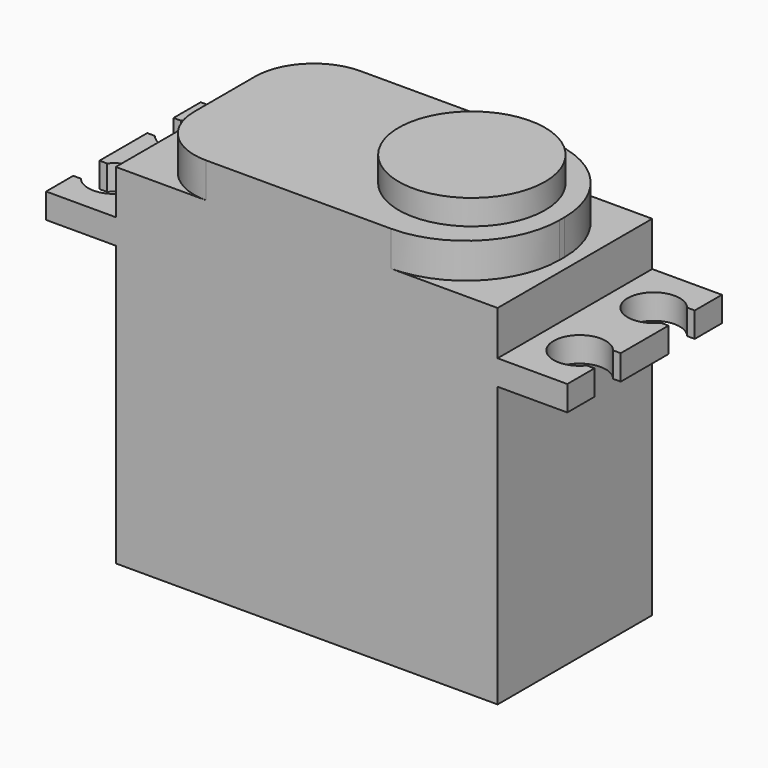
from build123d import *

# Parameters (mm, degrees)
F0_W      = 32.6
F0_H      = 29.8
F1_DEPTH  = 16.5
F2_W      = 28.8
F2_H      = 16.5
F3_DEPTH  = 3
F4_R      = 8
F5_R      = 5
F6_R      = 6.25
F7_DEPTH  = 2.14
F8_W      = 16.5
F8_H      = 2.14
F9_DEPTH  = 5.95
F11_DEPTH = 26.021


# Not quite as in the source:
# - a pattern or mirror of a feature is missing from the dataset's text; its kind, count and spacing are read off the source's solid


with BuildPart() as f1:
    # F0 (on Front) → F1 (new body)
    with BuildSketch(Plane.XZ):
        Rectangle(F0_W, F0_H)
    extrude(amount=F1_DEPTH)

    # F2 (on face) → F3 (join)
    with BuildSketch(Plane.XY.offset(14.9)):
        with Locations((0.8, -8.25)):
            Rectangle(F2_W, F2_H)
    extrude(amount=F3_DEPTH)

    # F4
    f4_edges = [f1.edges().sort_by_distance(p)[0] for p in [
        (15.2, -16.5, 16.4),
        (15.2, 0, 16.4),
    ]]
    fillet(f4_edges, radius=F4_R)

    # F5
    f5_edges = [f1.edges().sort_by_distance(p)[0] for p in [
        (-13.6, -16.5, 16.4),
        (-13.6, 0, 16.4),
    ]]
    fillet(f5_edges, radius=F5_R)

    # F6 (on face) → F7 (join)
    with BuildSketch(Plane.XY.offset(17.9)):
        with Locations((7.3, -8)):
            Circle(F6_R)
    extrude(amount=F7_DEPTH)

    # F8 (on face) → F9 (join)
    with BuildSketch(Plane.YZ.offset(16.3)):
        with Locations((-8.25, 10.05)):
            Rectangle(F8_W, F8_H)
    f9 = extrude(amount=F9_DEPTH)

    # F9_copies: F9 across plane
    add(f9.mirror(Plane(origin=(0, 0, 0), x_dir=(0, 0, -1), z_dir=(-1, 0, 0))))

    # F10 (on face) → F11 (cut, through all)
    with BuildSketch(Plane.XY.offset(11.12)):
        with BuildLine():
            ThreePointArc((21.5993423606, -5.7), (21.9674283959, -5.0425760055), (22.095, -4.3))
            ThreePointArc((22.095, -4.3), (21.9674283959, -3.5574239945), (21.5993423606, -2.9))
            Line((21.5993423606, -2.9), (21.5993423606, -5.7))
        make_face()
        with BuildLine():
            ThreePointArc((21.5993423606, -2.9), (21.9674283959, -3.5574239945), (22.095, -4.3))
            ThreePointArc((22.095, -4.3), (21.9674283959, -5.0425760055), (21.5993423606, -5.7))
            Line((21.5993423606, -5.7), (22.25, -5.7))
            Line((22.25, -5.7), (22.25, -2.9))
            Line((22.25, -2.9), (21.5993423606, -2.9))
        make_face()
        with BuildLine():
            Line((21.5993423606, -5.7), (21.5993423606, -2.9))
            ThreePointArc((21.5993423606, -2.9), (17.645, -4.3), (21.5993423606, -5.7))
        make_face()
        with BuildLine():
            ThreePointArc((21.5993423606, -13.6), (21.9674283959, -12.9425760055), (22.095, -12.2))
            ThreePointArc((22.095, -12.2), (21.9674283959, -11.4574239945), (21.5993423606, -10.8))
            Line((21.5993423606, -10.8), (21.5993423606, -13.6))
        make_face()
        with BuildLine():
            ThreePointArc((21.5993423606, -10.8), (21.9674283959, -11.4574239945), (22.095, -12.2))
            ThreePointArc((22.095, -12.2), (21.9674283959, -12.9425760055), (21.5993423606, -13.6))
            Line((21.5993423606, -13.6), (22.25, -13.6))
            Line((22.25, -13.6), (22.25, -10.8))
            Line((22.25, -10.8), (21.5993423606, -10.8))
        make_face()
        with BuildLine():
            Line((21.5993423606, -13.6), (21.5993423606, -10.8))
            ThreePointArc((21.5993423606, -10.8), (17.645, -12.2), (21.5993423606, -13.6))
        make_face()
    f11 = extrude(amount=-F11_DEPTH, mode=Mode.SUBTRACT)

    # F11_copies: F11 across plane
    add(f11.mirror(Plane(origin=(0, 0, 0), x_dir=(0, 0, -1), z_dir=(-1, 0, 0))), mode=Mode.SUBTRACT)


solid = f1.part
